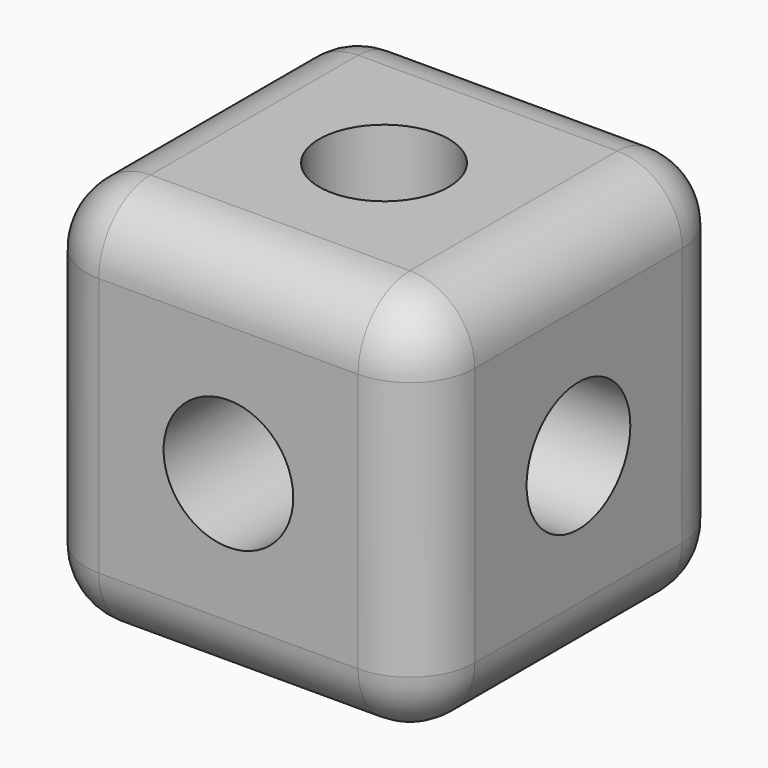
from build123d import *

# Parameters (mm, degrees)
F0_W         = 30
F0_H         = 30
F1_DEPTH     = 15
F2_R         = 5
F3_DEPTH     = 30.001
F4_R         = 5
F5_DEPTH     = 30.001
F6_R         = 5
F7_DEPTH     = 30.001
F8_R         = 5
F9_T1_DEPTH  = 20
F9_S5_W      = 5
F9_S5_H      = 5
F9_T6_DEPTH  = 5
F9_S11_W     = 5
F9_S11_H     = 5
F9_T12_DEPTH = 5


# Not quite as in the source:
# - a fillet or chamfer that OpenCascade refuses, or shapes differently, is made with other operations: its cross-section is extruded or revolved along the edge and cut away or added


with BuildPart() as f1:
    # F0 (on Top) → F1 (new body, symmetric)
    with BuildSketch(Plane.XY):
        Rectangle(F0_W, F0_H)
    extrude(amount=F1_DEPTH, both=True)

    # F2 (on face) → F3 (cut, through all)
    with BuildSketch(Plane.XY.offset(15)):
        Circle(F2_R)
    extrude(amount=-F3_DEPTH, mode=Mode.SUBTRACT)

    # F4 (on face) → F5 (cut, through all)
    with BuildSketch(Plane.YZ.offset(15)):
        Circle(F4_R)
    extrude(amount=-F5_DEPTH, mode=Mode.SUBTRACT)

    # F6 (on face) → F7 (cut, through all)
    with BuildSketch(Plane.XZ.offset(15)):
        Circle(F6_R)
    extrude(amount=-F7_DEPTH, mode=Mode.SUBTRACT)

    # F8
    f8_edges = [f1.edges().sort_by_distance(p)[0] for p in [
        (15, 0, 15),
        (0, 15, 15),
        (0, -15, 15),
        (-15, 0, 15),
        (-15, 15, 0),
        (15, -15, 0),
        (0, -15, -15),
        (-15, 0, -15),
        (15, 15, 0),
        (15, 0, -15),
        (-15, -15, 0),
    ]]
    fillet(f8_edges, radius=F8_R)

    # F9: fillet of radius 5 on 1 edges, made by hand

    # F9_s2 → F9_t1 (cut)
    with BuildSketch(Plane.YZ.offset(-10)):
        with BuildLine():
            ThreePointArc((15, -10), (13.5355339059, -13.5355339059), (10, -15))
            Line((10, -15), (15, -15))
            Line((15, -15), (15, -10))
        make_face()
    extrude(amount=F9_T1_DEPTH, mode=Mode.SUBTRACT)


with BuildPart() as f9_tool4:
    # F9_s5 → F9_t6 (new body)
    with BuildSketch(Plane.XZ.offset(-10)):
        with Locations((12.5, -12.5)):
            Rectangle(F9_S5_W, F9_S5_H)
    extrude(amount=-F9_T6_DEPTH)

    # F9_s7 → F9_t8 (revolve, cut)
    with BuildSketch(Plane(origin=(10, 10, -10), x_dir=(-0.7071067812, 0, 0.7071067812), z_dir=(-0.7071067812, 0, -0.7071067812))):
        with BuildLine():
            ThreePointArc((0, -5), (5, 0), (0, 5))
            Line((0, 5), (0, -5))
        make_face()
    revolve(axis=Axis((10, 10, -10), (0, 1, 0)), mode=Mode.SUBTRACT)


with BuildPart() as f1_1:
    add(f1.part)

    # F9_t3: cut F9_tool4
    add(f9_tool4.part, mode=Mode.SUBTRACT)


with BuildPart() as f9_tool10:
    # F9_s11 → F9_t12 (new body)
    with BuildSketch(Plane.XZ.offset(-10)):
        with Locations((-12.5, -12.5)):
            Rectangle(F9_S11_W, F9_S11_H)
    extrude(amount=-F9_T12_DEPTH)

    # F9_s13 → F9_t14 (revolve, cut)
    with BuildSketch(Plane(origin=(-10, 10, -10), x_dir=(0.7071067812, 0, 0.7071067812), z_dir=(-0.7071067812, 0, 0.7071067812))):
        with BuildLine():
            ThreePointArc((0, -5), (5, 0), (0, 5))
            Line((0, 5), (0, -5))
        make_face()
    revolve(axis=Axis((-10, 10, -10), (0, 1, 0)), mode=Mode.SUBTRACT)


with BuildPart() as f1_2:
    add(f1_1.part)

    # F9_t9: cut F9_tool10
    add(f9_tool10.part, mode=Mode.SUBTRACT)


solid = f1_2.part
